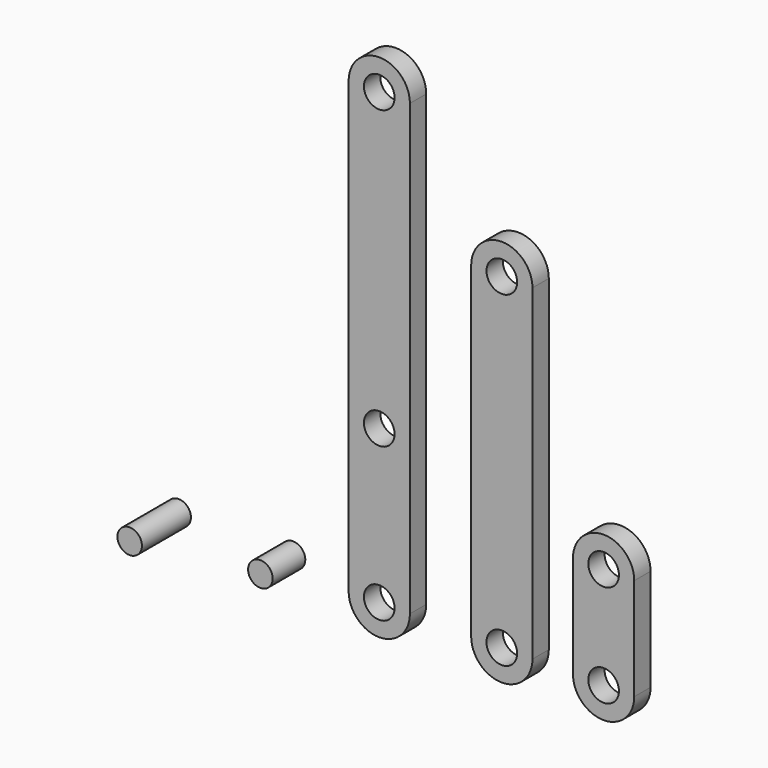
from build123d import *

# Parameters (mm, degrees)
F1_R      = 7.5
F2_DEPTH  = 10
F3_R      = 7.5
F4_DEPTH  = 10
F5_R      = 7.5
F6_DEPTH  = 10
F7_R      = 6
F8_DEPTH  = 20
F9_R      = 6
F10_DEPTH = 30


with BuildPart() as f2:
    # F1 (on Front) → F2 (new body)
    with BuildSketch(Plane.XZ):
        with BuildLine():
            Line((-15, 50), (-15, 0))
            ThreePointArc((-15, 0), (0, -15), (15, 0))
            Line((15, 0), (15, 50))
            ThreePointArc((15, 50), (0, 65), (-15, 50))
        make_face()
        Circle(F1_R, mode=Mode.SUBTRACT)
        with Locations((0, 50)):
            Circle(F1_R, mode=Mode.SUBTRACT)
    extrude(amount=F2_DEPTH)


with BuildPart() as f4:
    # F3 (on Front) → F4 (new body)
    with BuildSketch(Plane.XZ):
        with BuildLine():
            Line((-64.8352653698, 160), (-64.8352653698, 0))
            ThreePointArc((-64.8352653698, 0), (-49.8352653698, -15), (-34.8352653698, 0))
            Line((-34.8352653698, 0), (-34.8352653698, 160))
            ThreePointArc((-34.8352653698, 160), (-49.8352653698, 175), (-64.8352653698, 160))
        make_face()
        with Locations((-49.8352653698, 0)):
            Circle(F3_R, mode=Mode.SUBTRACT)
        with Locations((-49.8352653698, 160)):
            Circle(F3_R, mode=Mode.SUBTRACT)
    extrude(amount=F4_DEPTH)


with BuildPart() as f6:
    # F5 (on Front) → F6 (new body)
    with BuildSketch(Plane.XZ):
        with BuildLine():
            Line((-124.8352653698, 220), (-124.8352653698, 0))
            ThreePointArc((-124.8352653698, 0), (-109.8352653698, -15), (-94.8352653698, 0))
            Line((-94.8352653698, 0), (-94.8352653698, 220))
            ThreePointArc((-94.8352653698, 220), (-109.8352653698, 235), (-124.8352653698, 220))
        make_face()
        with BuildLine():
            ThreePointArc((-109.8352653698, 7.5), (-104.5319645109, 5.3033008589), (-102.3352653698, 0))
            ThreePointArc((-102.3352653698, 0), (-115.1385662287, -5.3033008589), (-109.8352653698, 7.5))
        make_face(mode=Mode.SUBTRACT)
        with BuildLine():
            ThreePointArc((-102.3352653698, 75), (-104.5319645109, 69.6966991411), (-109.8352653698, 67.5))
            ThreePointArc((-109.8352653698, 67.5), (-115.1385662287, 80.3033008589), (-102.3352653698, 75))
        make_face(mode=Mode.SUBTRACT)
        with Locations((-109.8352653698, 220)):
            Circle(F5_R, mode=Mode.SUBTRACT)
    extrude(amount=F6_DEPTH)


with BuildPart() as f8:
    # F7 (on Front) → F8 (new body)
    with BuildSketch(Plane.XZ):
        with Locations((-160.0444316864, 0)):
            Circle(F7_R)
    extrude(amount=F8_DEPTH)


with BuildPart() as f10:
    # F9 (on Front) → F10 (new body)
    with BuildSketch(Plane.XZ):
        with Locations((-216.0444316864, 0)):
            Circle(F9_R)
    extrude(amount=F10_DEPTH)


solid = Compound([f2.part, f4.part, f6.part, f8.part, f10.part])
